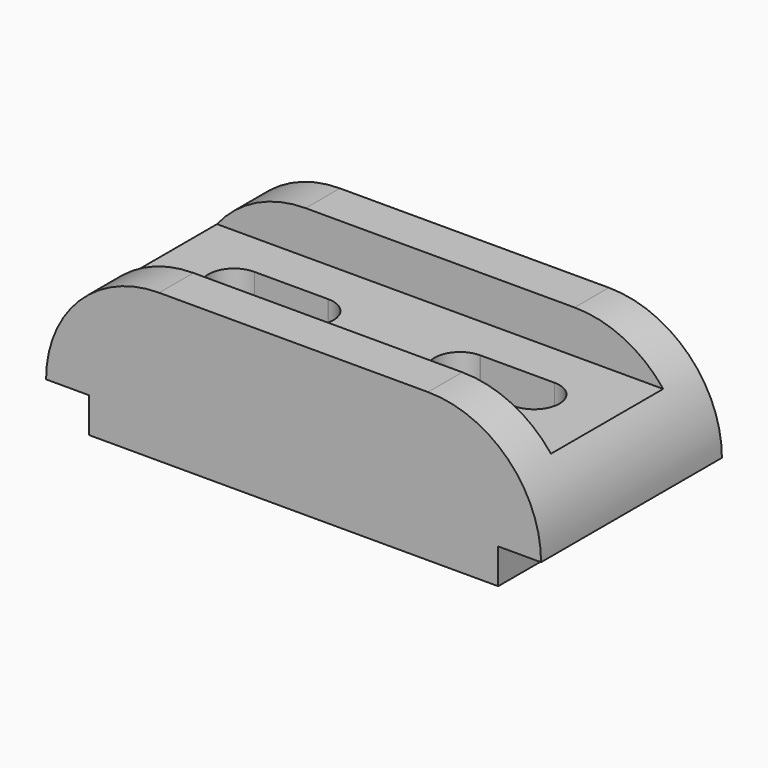
from build123d import *

# Parameters (mm, degrees)
F0_W     = 3225.8
F0_H     = 965.2
F1_DEPTH = 1473.2
F3_DEPTH = 965.201
F4_W     = 914.4
F4_H     = 279.4
F5_DEPTH = 3225.801
F6_W     = 279.4
F6_H     = 228.6
F7_DEPTH = 1473.201
F8_R     = 736.59999


# Not quite as in the source:
# - a fillet or chamfer is up to 0.001 mm smaller than in the source, because OpenCascade refuses the exact size


with BuildPart() as f1:
    # F0 (on Front) → F1 (new body)
    with BuildSketch(Plane.XZ):
        Rectangle(F0_W, F0_H)
    extrude(amount=F1_DEPTH)

    # F2 (on face) → F3 (cut, through all)
    with BuildSketch(Plane.XY.offset(482.6)):
        with BuildLine():
            Line((-495.6148372224, -571.5003001895), (-977.5851627776, -571.5003001895))
            ThreePointArc((-977.5851627776, -571.5003001895), (-1142.9401608263, -741.0446950901), (-968.6994670012, -901.4434414605))
            Line((-968.6994670012, -901.4434414605), (-504.5005329988, -901.4434414605))
            Line((-504.5005329988, -901.4434414605), (-486.0994670012, -901.4434414605))
            ThreePointArc((-486.0994670012, -901.4434414605), (-330.2598391737, -732.15530491), (-494.9851627776, -571.5003001895))
            Line((-494.9851627776, -571.5003001895), (-495.6148372224, -571.5003001895))
        make_face()
        with BuildLine():
            ThreePointArc((-494.9851627776, -571.5003001895), (-495.3, -571.5), (-495.6148372224, -571.5003001895))
            Line((-495.6148372224, -571.5003001895), (-494.9851627776, -571.5003001895))
        make_face()
        with BuildLine():
            Line((-486.0994670012, -901.4434414605), (-504.5005329988, -901.4434414605))
            ThreePointArc((-504.5005329988, -901.4434414605), (-495.3, -901.7), (-486.0994670012, -901.4434414605))
        make_face()
        with BuildLine():
            ThreePointArc((968.6994670012, -901.4434414605), (1142.9401608263, -741.0446950901), (977.5851627776, -571.5003001895))
            Line((977.5851627776, -571.5003001895), (495.6148372224, -571.5003001895))
            Line((495.6148372224, -571.5003001895), (494.9851627776, -571.5003001895))
            ThreePointArc((494.9851627776, -571.5003001895), (330.2598391737, -732.15530491), (486.0994670012, -901.4434414605))
            Line((486.0994670012, -901.4434414605), (504.5005329988, -901.4434414605))
            Line((504.5005329988, -901.4434414605), (968.6994670012, -901.4434414605))
        make_face()
        with BuildLine():
            Line((494.9851627776, -571.5003001895), (495.6148372224, -571.5003001895))
            ThreePointArc((495.6148372224, -571.5003001895), (495.3, -571.5), (494.9851627776, -571.5003001895))
        make_face()
        with BuildLine():
            ThreePointArc((486.0994670012, -901.4434414605), (495.3, -901.7), (504.5005329988, -901.4434414605))
            Line((504.5005329988, -901.4434414605), (486.0994670012, -901.4434414605))
        make_face()
    extrude(amount=-F3_DEPTH, mode=Mode.SUBTRACT)

    # F4 (on face) → F5 (cut, through all)
    with BuildSketch(Plane.YZ.offset(1612.9)):
        with Locations((-736.6, 342.9)):
            Rectangle(F4_W, F4_H)
    extrude(amount=-F5_DEPTH, mode=Mode.SUBTRACT)

    # F6 (on face) → F7 (cut, through all)
    with BuildSketch(Plane.XZ.offset(1473.2)):
        with Locations((-1473.2, -368.3)):
            Rectangle(F6_W, F6_H)
        with Locations((1473.2, -368.3)):
            Rectangle(F6_W, F6_H)
    extrude(amount=-F7_DEPTH, mode=Mode.SUBTRACT)

    # F8 (radius 736.6 in the source; OpenCascade refuses exactly that, so slightly less here)
    f8_edges = [f1.edges().sort_by_distance(p)[0] for p in [
        (-1612.9, -1333.5, 482.6),
        (1612.9, -1333.5, 482.6),
    ]]
    fillet(f8_edges, radius=F8_R)


solid = f1.part
